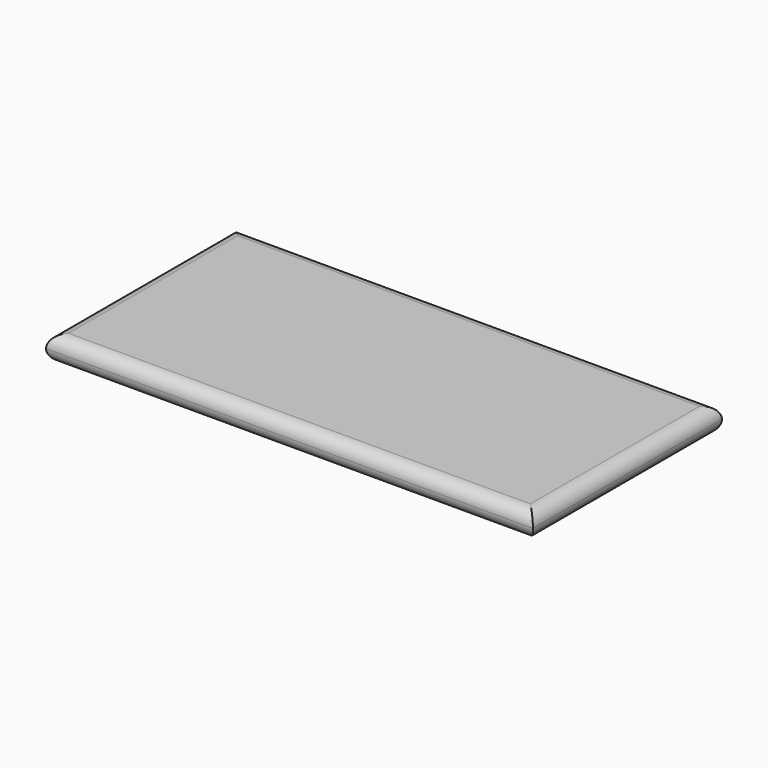
from build123d import *

# Parameters (mm, degrees)
F0_W     = 138.29
F0_H     = 67.12
F1_DEPTH = 7.1
F2_R     = 3.54999


# Not quite as in the source:
# - a fillet or chamfer is up to 0.001 mm smaller than in the source, because OpenCascade refuses the exact size


with BuildPart() as f1:
    # F0 (on Top) → F1 (new body)
    with BuildSketch(Plane.XY):
        Rectangle(F0_W, F0_H)
    extrude(amount=F1_DEPTH)

    # F2 (radius 3.55 in the source; OpenCascade refuses exactly that, so slightly less here)
    f2_edges = [f1.edges().sort_by_distance(p)[0] for p in [
        (0, -33.56, 0),
        (69.145, 0, 7.1),
        (69.145, 0, 0),
        (0, 33.56, 7.1),
        (0, 33.56, 0),
        (-69.145, 0, 7.1),
        (-69.145, 0, 0),
        (0, -33.56, 7.1),
    ]]
    fillet(f2_edges, radius=F2_R)


solid = f1.part
